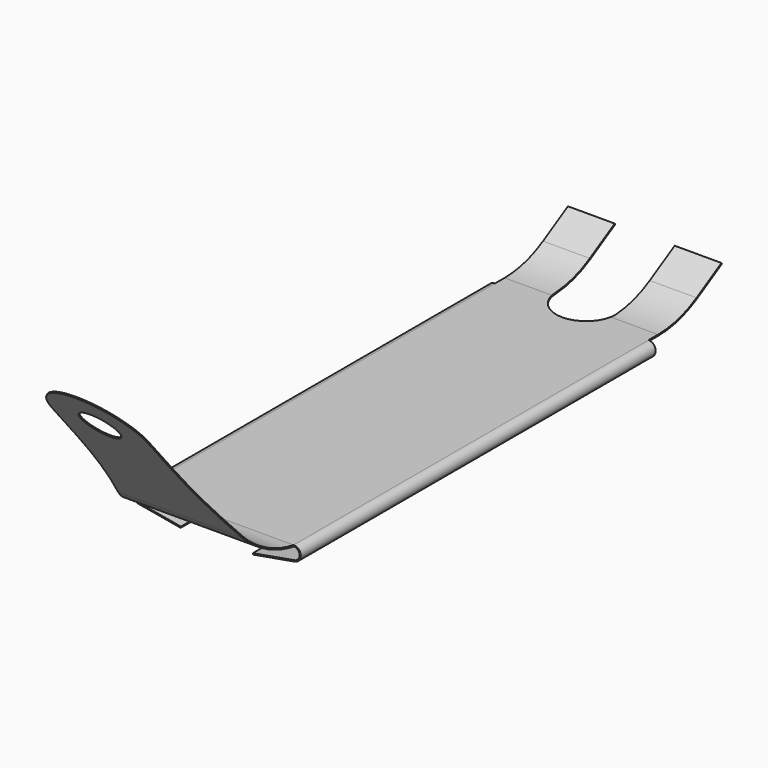
from build123d import *

# Parameters (mm, degrees)
F1_DEPTH = 64
F3_DEPTH = 370
F6_DEPTH = 500
F8_R     = 15.9
F9_DEPTH = 600


# Not quite as in the source:
# - a feature names something its author has since deleted; it is built from what else it names


with BuildPart() as f1:
    # F0 (on Right) → F1 (new body, symmetric)
    with BuildSketch(Plane.YZ):
        with BuildLine():
            Line((380, 0), (0, 0))
            ThreePointArc((0, 0), (-20.7082948253, 4.5909184352), (-37.5361777128, 17.5034071254))
            Line((-37.5361777128, 17.5034071254), (-121, 116.9717171877))
            Line((-121, 116.9717171877), (-187.1849916482, 195.8479187603))
            Line((-187.1849916482, 195.8479187603), (-187.8376952929, 195.0700568469))
            Line((-187.8376952929, 195.0700568469), (-128.3694552412, 124.1985681201))
            Line((-128.3694552412, 124.1985681201), (-38.3022221559, 16.8606195157))
            ThreePointArc((-38.3022221559, 16.8606195157), (-21.130913087, 3.6846106482), (0, -1))
            Line((0, -1), (380, -1))
            ThreePointArc((380, -1), (400.9643426533, 1.7600080706), (420.5, 9.8519422935))
            Line((420.5, 9.8519422935), (446.4807621135, 24.8519422935))
            Line((446.4807621135, 24.8519422935), (445.9807621135, 25.7179676972))
            Line((445.9807621135, 25.7179676972), (420, 10.7179676972))
            ThreePointArc((420, 10.7179676972), (400.7055236082, 2.7259338969), (380, 0))
        make_face()
    extrude(amount=F1_DEPTH, both=True)

    # F2 (on Front) → F3 (join)
    with BuildSketch(Plane.XZ):
        with BuildLine():
            ThreePointArc((65.041889066, -11.9088465181), (69.9771681886, -5.4770655435), (64, 0))
            Line((64, 0), (-64, 0))
            ThreePointArc((-64, 0), (-69.9771681886, -5.4770655435), (-65.041889066, -11.9088465181))
            Line((-65.041889066, -11.9088465181), (-30.1606090351, -18.0593573092))
            Line((-30.1606090351, -18.0593573092), (-29.9869608574, -17.0745495562))
            Line((-29.9869608574, -17.0745495562), (-64.8682408883, -10.9240387651))
            ThreePointArc((-64.8682408883, -10.9240387651), (-68.9809734905, -5.5642212863), (-64, -1))
            Line((-64, -1), (64, -1))
            ThreePointArc((64, -1), (68.9809734905, -5.5642212863), (64.8682408883, -10.9240387651))
            Line((64.8682408883, -10.9240387651), (29.9869608574, -17.0745495562))
            Line((29.9869608574, -17.0745495562), (30.1606090351, -18.0593573092))
            Line((30.1606090351, -18.0593573092), (65.041889066, -11.9088465181))
        make_face()
    extrude(amount=-F3_DEPTH)

    # F5 (on offset) → F6 (cut)
    with BuildSketch(Plane.XY.offset(400)):
        with BuildLine():
            Line((-25, 446.4807621135), (-25, 385))
            ThreePointArc((-25, 385), (0, 360), (25, 385))
            Line((25, 385), (25, 446.4807621135))
            Line((25, 446.4807621135), (-25, 446.4807621135))
        make_face()
    extrude(amount=-F6_DEPTH, mode=Mode.SUBTRACT)

    # F8 (on offset) → F9 (cut)
    with BuildSketch(Plane(origin=(0, 369.6138337955, 310.1428316158), x_dir=(-1, 0, 0), z_dir=(0, 0.7660444431, 0.6427876097))):
        with Locations((0, 167.3828347258)):
            Circle(F8_R)
        with BuildLine():
            ThreePointArc((-40, 167.3828347258), (0, 207.3828347258), (40, 167.3828347258))
            Line((40, 167.3828347258), (40, 127.3828347258))
            ThreePointArc((40, 127.3828347258), (46.052321998, 62.5708246837), (64, 0))
            Line((64, 0), (64, 37.5361777128))
            Line((64, 37.5361777128), (64, 270.3484032135))
            Line((64, 270.3484032135), (-64, 270.3484032135))
            Line((-64, 270.3484032135), (-64, 37.5361777128))
            Line((-64, 37.5361777128), (-64, 0))
            ThreePointArc((-64, 0), (-46.052321998, 62.5708246837), (-40, 127.3828347258))
            Line((-40, 127.3828347258), (-40, 167.3828347258))
        make_face()
    extrude(amount=-F9_DEPTH, mode=Mode.SUBTRACT)


solid = f1.part
